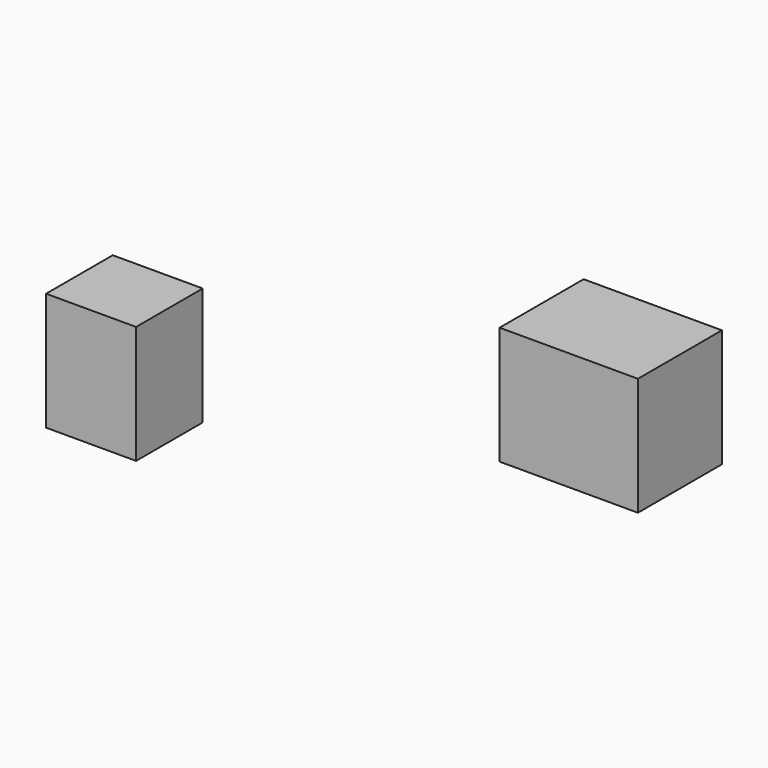
from build123d import *

# Parameters (mm, degrees)
F2_W     = 1830.7656049728
F2_H     = 1695.1532363892
F3_DEPTH = 2400
F2_W_2   = 2813.9543533325
F2_H_2   = 2135.8923912048


# Not quite as in the source:
# - the program builds the solid bodies; features that only make, move or delete a surface that nothing else refers to are left out


with BuildPart() as f3:
    # F2 (on Top) → F3 (new body)
    with BuildSketch(Plane.XY):
        with Locations((-915.3828024864, -10152.4233818054)):
            Rectangle(F2_W, F2_H)
    extrude(amount=F3_DEPTH)


with BuildPart() as f3b:
    # F2 (on Top) → F3, piece 2 (new body)
    with BuildSketch(Plane.XY):
        with Locations((5933.0353736877, -6343.9795970917)):
            Rectangle(F2_W_2, F2_H_2)
    extrude(amount=F3_DEPTH)


solid = Compound([f3.part, f3b.part])
